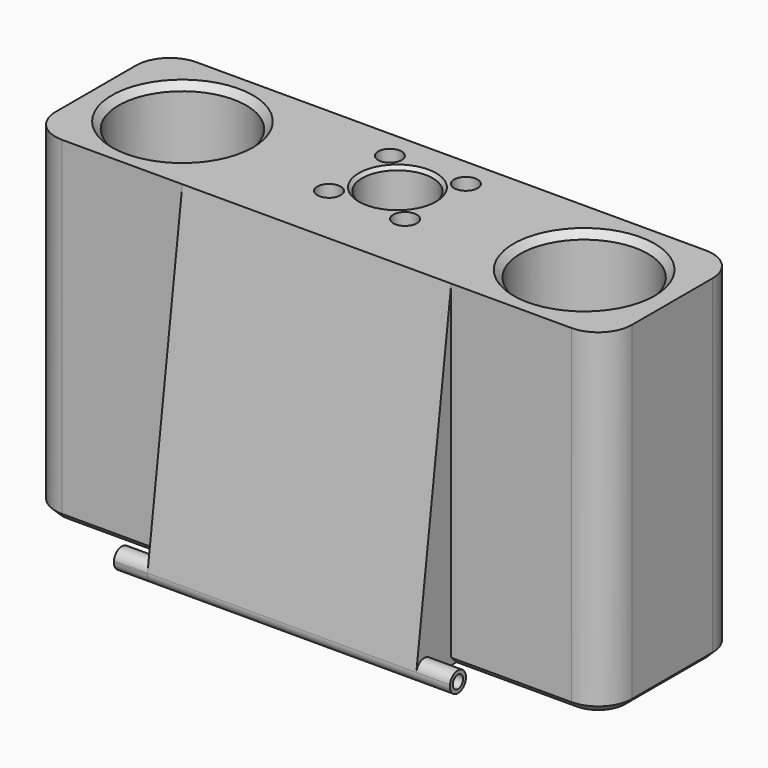
from build123d import *
from build123d import SkipClean  # not in build123d's __all__

# Parameters (mm, degrees)
F0_W      = 85.7687139645
F0_H      = 25
F0_R      = 9.5
F0_R_2    = 5.25
F1_DEPTH  = 50
F3_R      = 0.95
F4_DEPTH  = 20
F5_R      = 0.95
F6_DEPTH  = 5
F7_R      = 0.95
F8_DEPTH  = 5
F9_R      = 1.75
F10_DEPTH = 50
F11_R     = 5
F12_SIZE  = 1
F13_SIZE  = 0.5
F14_SIZE  = 1


# Not quite as in the source:
# - after a boolean that leaves OpenCascade's solid faulty, fix() repairs it


with BuildPart() as f1:
    # F0 (on Top) → F1 (new body)
    with BuildSketch(Plane.XY):
        with Locations((0, 168.5)):
            Rectangle(F0_W, F0_H)
        with Locations((-29.8843569823, 168.3684210526)):
            Circle(F0_R, mode=Mode.SUBTRACT)
        with Locations((29.8843569823, 168.3684210526)):
            Circle(F0_R, mode=Mode.SUBTRACT)
        with Locations((0, 171)):
            Circle(F0_R_2, mode=Mode.SUBTRACT)
    extrude(amount=F1_DEPTH)

    # F3 (on mid) → F4 (join, symmetric)
    with BuildSketch(Plane.YZ):
        with BuildLine():
            Line((156, 50), (149.5133467482, 1.6996549744))
            ThreePointArc((149.5133467482, 1.6996549744), (149.8709556117, 0.5124480929), (151, 0))
            Line((151, 0), (156, 0))
            Line((156, 0), (156, 50))
        make_face()
        with Locations((151, 1.5)):
            Circle(F3_R, mode=Mode.SUBTRACT)
    extrude(amount=F4_DEPTH, both=True)

    # F5 (on face) → F6 (join)
    with BuildSketch(Plane.YZ.offset(20)):
        with BuildLine():
            ThreePointArc((151, 0), (152.0606601718, 0.4393398282), (152.5, 1.5))
            ThreePointArc((152.5, 1.5), (151.100050293, 2.9966595935), (149.5133467482, 1.6996549744))
            ThreePointArc((149.5133467482, 1.6996549744), (149.8709556117, 0.5124480929), (151, 0))
        make_face()
        with Locations((151, 1.5)):
            Circle(F5_R, mode=Mode.SUBTRACT)
    extrude(amount=F6_DEPTH)

    # F7 (on face) → F8 (join)
    with BuildSketch(Plane(origin=(-20, 0, 0), x_dir=(0, -1, 0), z_dir=(-1, 0, 0))):
        with BuildLine():
            ThreePointArc((-151, 0), (-149.9393398282, 0.4393398282), (-149.5, 1.5))
            ThreePointArc((-149.5, 1.5), (-149.5033404065, 1.600050293), (-149.5133467482, 1.6996549744))
            ThreePointArc((-149.5133467482, 1.6996549744), (-152.1290443883, 2.4875519071), (-151, 0))
        make_face()
        with Locations((-151, 1.5)):
            Circle(F7_R, mode=Mode.SUBTRACT)
    with SkipClean():  # cleaning this boolean's faces spoils the solid; the shape is the same uncleaned
        extrude(amount=F8_DEPTH)

    # F9 (on face) → F10 (cut, through all)
    with BuildSketch(Plane.XY.offset(50)):
        with Locations((5.6568542495, 176.6568542495)):
            Circle(F9_R)
        with Locations((-5.6568542495, 176.6568542495)):
            Circle(F9_R)
        with Locations((-5.6568542495, 165.3431457505)):
            Circle(F9_R)
        with Locations((5.6568542495, 165.3431457505)):
            Circle(F9_R)
    extrude(amount=-F10_DEPTH, mode=Mode.SUBTRACT)

    add(f1.part.fix(), mode=Mode.REPLACE)

    # F11
    f11_edges = [f1.edges().sort_by_distance(p)[0] for p in [
        (42.884357, 156, 25),
        (42.884357, 181, 25),
        (-42.884357, 181, 25),
        (-42.884357, 156, 25),
    ]]
    fillet(f11_edges, radius=F11_R)

    # F12
    f12_edges = [f1.edges().sort_by_distance(p)[0] for p in [
        (20.384357, 168.368421, 50),
        (-39.384357, 168.368421, 50),
        (20.384357, 168.368421, 0),
        (-39.384357, 168.368421, 0),
    ]]
    chamfer(f12_edges, length=F12_SIZE)

    # F13
    f13_edges = [f1.edges().sort_by_distance(p)[0] for p in [
        (-5.25, 171, 50),
        (-5.25, 171, 0),
    ]]
    chamfer(f13_edges, length=F13_SIZE)

    # F14
    f14_edges = [f1.edges().sort_by_distance(p)[0] for p in [
        (-28.942178, 156, 0),
        (-41.419891, 157.464466, 0),
        (42.884357, 168.5, 0),
        (41.419891, 157.464466, 0),
        (41.419891, 179.535534, 0),
        (28.942178, 156, 0),
        (0, 181, 0),
        (-41.419891, 179.535534, 0),
        (-42.884357, 168.5, 0),
    ]]
    chamfer(f14_edges, length=F14_SIZE)


solid = f1.part
